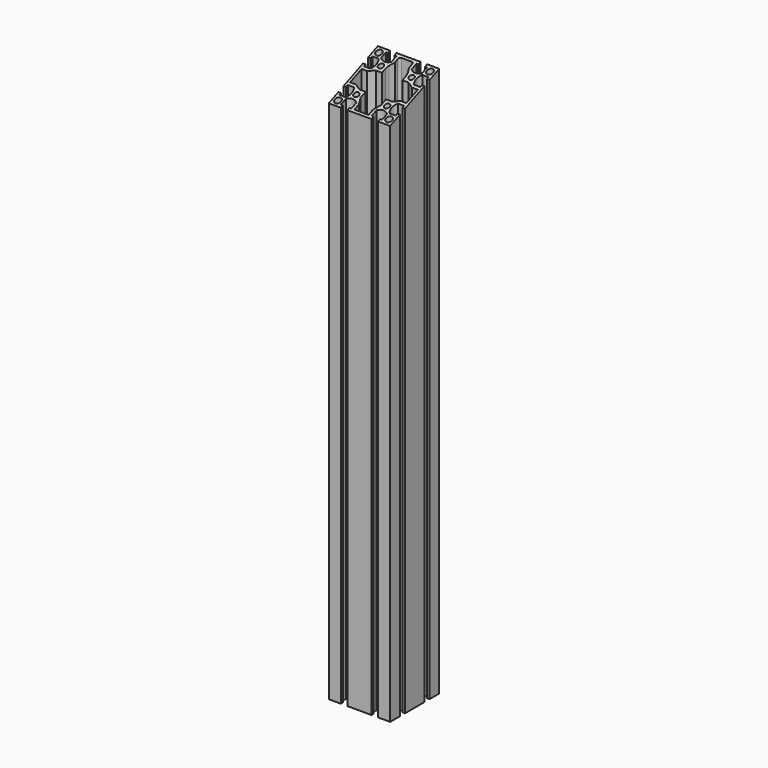
from build123d import *

# Parameters (mm, degrees)
F0_R          = 3
F0_R_2        = 2.5
F1_DEPTH      = 537.86
F2_R          = 2
F3_R          = 7
F5_DEPTH      = 30
F5_DEPTH_BACK = 30


# Not quite as in the source:
# - a feature names something its author has since deleted; it is built from what else it names


with BuildPart() as f1:
    # F0 (on Top) → F1 (new body)
    with BuildSketch(Plane.XY):
        with BuildLine():
            Line((18.15, -30), (30, -30))
            Line((30, -30), (30, -18.15))
            Line((30, -18.15), (27.5, -18.15))
            Line((27.5, -18.15), (27.5, -20.15))
            Line((27.5, -20.15), (21.5477069044, -20.15))
            ThreePointArc((21.5477069044, -20.15), (19.5, -15), (21.5477069044, -9.85))
            Line((21.5477069044, -9.85), (27.5, -9.85))
            Line((27.5, -9.85), (27.5, -11.85))
            Line((27.5, -11.85), (30, -11.85))
            Line((30, -11.85), (30, 11.85))
            Line((30, 11.85), (27.5, 11.85))
            Line((27.5, 11.85), (27.5, 9.85))
            Line((27.5, 9.85), (21.5477069044, 9.85))
            ThreePointArc((21.5477069044, 9.85), (19.5, 15), (21.5477069044, 20.15))
            Line((21.5477069044, 20.15), (27.5, 20.15))
            Line((27.5, 20.15), (27.5, 18.15))
            Line((27.5, 18.15), (30, 18.15))
            Line((30, 18.15), (30, 30))
            Line((30, 30), (18.15, 30))
            Line((18.15, 30), (18.15, 27.5))
            Line((18.15, 27.5), (20.15, 27.5))
            Line((20.15, 27.5), (20.15, 21.5477069044))
            ThreePointArc((20.15, 21.5477069044), (15, 19.5), (9.85, 21.5477069044))
            Line((9.85, 21.5477069044), (9.85, 27.5))
            Line((9.85, 27.5), (11.85, 27.5))
            Line((11.85, 27.5), (11.85, 30))
            Line((11.85, 30), (-11.85, 30))
            Line((-11.85, 30), (-11.85, 27.5))
            Line((-11.85, 27.5), (-9.85, 27.5))
            Line((-9.85, 27.5), (-9.85, 21.5477069044))
            ThreePointArc((-9.85, 21.5477069044), (-15, 19.5), (-20.15, 21.5477069044))
            Line((-20.15, 21.5477069044), (-20.15, 27.5))
            Line((-20.15, 27.5), (-18.15, 27.5))
            Line((-18.15, 27.5), (-18.15, 30))
            Line((-18.15, 30), (-30, 30))
            Line((-30, 30), (-30, 18.15))
            Line((-30, 18.15), (-27.5, 18.15))
            Line((-27.5, 18.15), (-27.5, 20.15))
            Line((-27.5, 20.15), (-21.5477069044, 20.15))
            ThreePointArc((-21.5477069044, 20.15), (-19.5, 15), (-21.5477069044, 9.85))
            Line((-21.5477069044, 9.85), (-27.5, 9.85))
            Line((-27.5, 9.85), (-27.5, 11.85))
            Line((-27.5, 11.85), (-30, 11.85))
            Line((-30, 11.85), (-30, -11.85))
            Line((-30, -11.85), (-27.5, -11.85))
            Line((-27.5, -11.85), (-27.5, -9.85))
            Line((-27.5, -9.85), (-21.5477069044, -9.85))
            ThreePointArc((-21.5477069044, -9.85), (-19.5, -15), (-21.5477069044, -20.15))
            Line((-21.5477069044, -20.15), (-27.5, -20.15))
            Line((-27.5, -20.15), (-27.5, -18.15))
            Line((-27.5, -18.15), (-30, -18.15))
            Line((-30, -18.15), (-30, -30))
            Line((-30, -30), (-18.15, -30))
            Line((-18.15, -30), (-18.15, -27.5))
            Line((-18.15, -27.5), (-20.15, -27.5))
            Line((-20.15, -27.5), (-20.15, -21.5477069044))
            ThreePointArc((-20.15, -21.5477069044), (-15, -19.5), (-9.85, -21.5477069044))
            Line((-9.85, -21.5477069044), (-9.85, -27.5))
            Line((-9.85, -27.5), (-11.85, -27.5))
            Line((-11.85, -27.5), (-11.85, -30))
            Line((-11.85, -30), (11.85, -30))
            Line((11.85, -30), (11.85, -27.5))
            Line((11.85, -27.5), (9.85, -27.5))
            Line((9.85, -27.5), (9.85, -21.5477069044))
            ThreePointArc((9.85, -21.5477069044), (15, -19.5), (20.15, -21.5477069044))
            Line((20.15, -21.5477069044), (20.15, -27.5))
            Line((20.15, -27.5), (18.15, -27.5))
            Line((18.15, -27.5), (18.15, -30))
        make_face()
        with Locations((-25, -25)):
            Circle(F0_R, mode=Mode.SUBTRACT)
        with Locations((-15, -15)):
            Circle(F0_R_2, mode=Mode.SUBTRACT)
        with Locations((25, -25)):
            Circle(F0_R, mode=Mode.SUBTRACT)
        with Locations((15, -15)):
            Circle(F0_R_2, mode=Mode.SUBTRACT)
        with Locations((-25, 25)):
            Circle(F0_R, mode=Mode.SUBTRACT)
        with Locations((-15, 15)):
            Circle(F0_R_2, mode=Mode.SUBTRACT)
        Polygon((-7, 22), (-7, 27.5), (0, 27.5), (7, 27.5), (7, 22), (10, 16), (10, 10), (16, 10), (22, 7), (27.5, 7), (27.5, 0), (27.5, -7), (22, -7), (16, -10), (10, -10), (10, -16), (7, -22), (7, -27.5), (0, -27.5), (-7, -27.5), (-7, -22), (-10, -16), (-10, -10), (-16, -10), (-22, -7), (-27.5, -7), (-27.5, 0), (-27.5, 7), (-22, 7), (-16, 10), (-10, 10), (-10, 16), align=None, mode=Mode.SUBTRACT)
        with Locations((15, 15)):
            Circle(F0_R_2, mode=Mode.SUBTRACT)
        with Locations((25, 25)):
            Circle(F0_R, mode=Mode.SUBTRACT)
    extrude(amount=F1_DEPTH)

    # F2
    f2_edges = [f1.edges().sort_by_distance(p)[0] for p in [
        (-7, 27.5, 268.93),
        (7, 27.5, 268.93),
    ]]
    fillet(f2_edges, radius=F2_R)

    # F3
    f3_edges = [f1.edges().sort_by_distance(p)[0] for p in [
        (-10, 16, 268.93),
        (10, 16, 268.93),
    ]]
    fillet(f3_edges, radius=F3_R)

    # F4 (on Right) → F5 (cut, two sides)
    with BuildSketch(Plane.YZ) as f5_sk:
        Polygon((-77.6874923482, 797.8406045251), (-234.1260457354, 733.041634034), (-126.4385533872, 473.061029509), (30, 537.86), align=None)
    extrude(amount=F5_DEPTH, mode=Mode.SUBTRACT)
    extrude(f5_sk.sketch, amount=-F5_DEPTH_BACK, mode=Mode.SUBTRACT)


solid = f1.part
